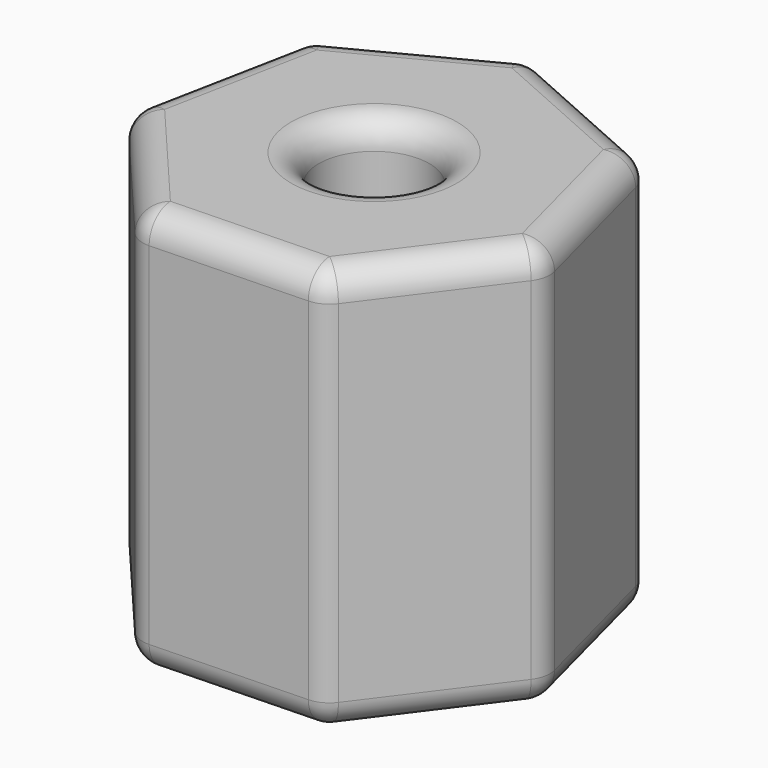
from build123d import *

# Parameters (mm, degrees)
F1_DEPTH       = 73.5
F3_D           = 20
F3_CBORE_D     = 20
F3_CBORE_DEPTH = 20
F4_R           = 5


# Not quite as in the source:
# - two fillets or chamfers of one size are made in one step


with BuildPart() as f1:
    # F0 (on Top) → F1 (new body)
    with BuildSketch(Plane.XY):
        Polygon((-1.1557375875, 37.9352838977), (-30.379589847, 22.7486706094), (-36.726991321, -9.568155636), (-15.4182192362, -34.6799655328), (17.5007864078, -33.6770540409), (37.2413429358, -7.3146339696), (28.9384086481, 24.5558546722), align=None)
    extrude(amount=F1_DEPTH)

    # F3 (through all)
    with Locations(Plane.XY.offset(73.5)):
        with Locations((0, 0)):
            CounterBoreHole(F3_D / 2, F3_CBORE_D / 2, F3_CBORE_DEPTH)

    # F4
    f4_edges = [f1.edges().sort_by_distance(p)[0] for p in [
        (-26.072605, -22.124061, 0),
        (-33.553291, 6.590257, 0),
        (-36.726991, -9.568156, 36.75),
        (-15.418219, -34.679966, 36.75),
        (-33.553291, 6.590257, 73.5),
        (-26.072605, -22.124061, 73.5),
        (-15.767664, 30.341977, 73.5),
        (-30.37959, 22.748671, 36.75),
        (-1.155738, 37.935284, 36.75),
        (28.938409, 24.555855, 36.75),
        (13.891336, 31.245569, 73.5),
        (33.089876, 8.62061, 73.5),
        (13.891336, 31.245569, 0),
        (33.089876, 8.62061, 0),
        (1.041284, -34.17851, 0),
        (27.371065, -20.495844, 0),
        (17.500786, -33.677054, 36.75),
        (37.241343, -7.314634, 36.75),
        (1.041284, -34.17851, 73.5),
        (27.371065, -20.495844, 73.5),
        (-15.767664, 30.341977, 0),
        (-10, 0, 0),
        (-10, 0, 73.5),
    ]]
    fillet(f4_edges, radius=F4_R)


solid = f1.part
